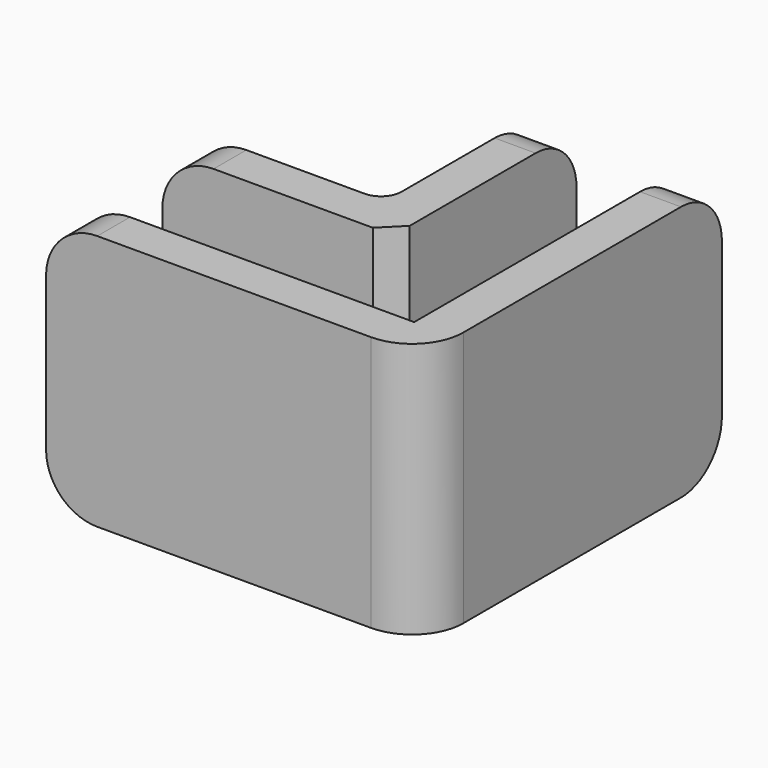
from build123d import *
from build123d import SkipClean  # not in build123d's __all__

# Parameters (mm, degrees)
F1_DEPTH       = 2
F2_DEPTH       = 25
F3_T1_DEPTH    = 29
F3_T3_DEPTH    = 29
F3_T5_DEPTH    = 29
F3_T7_DEPTH    = 29
F3_T9_DEPTH    = 43.2
F3_T11_DEPTH   = 43.2
F3_T13_DEPTH   = 50
F4_R           = 2
F5_SIZE        = 2
F7_D           = 3.3
F7_CSINK_D     = 6
F7_CSINK_ANGLE = 90


# Not quite as in the source:
# - a fillet or chamfer that OpenCascade refuses, or shapes differently, is made with other operations: its cross-section is extruded or revolved along the edge and cut away or added
# - a feature names something its author has since deleted; it is built from what else it names


with BuildPart() as f1:
    # F0 (on Top) → F1 (new body)
    with BuildSketch(Plane.XY):
        Polygon((5.1, 0), (5.1, 10.2), (5.1, 32.5735770881), (-5.1, 32.5735770881), (-5.1, 10.2), (-27.6520505063, 10.2), (-27.6520505063, 0), (0, 0), align=None)
        Polygon((5.1, 32.5735770881), (5.1, 10.2), (5.1, 0), (0, 0), (-27.6520505063, 0), (-27.6520505063, -4), (0, -4), (9.1, -4), (9.1, 32.5735770881), align=None)
        Polygon((-5.1, 10.2), (-5.1, 32.5735770881), (-9.1, 32.5735770881), (-9.1, 14.2), (-27.6520505063, 14.2), (-27.6520505063, 10.2), align=None)
    extrude(amount=F1_DEPTH)

    # F0 (on Top) → F2 (join)
    with BuildSketch(Plane.XY):
        Polygon((-5.1, 10.2), (-5.1, 32.5735770881), (-9.1, 32.5735770881), (-9.1, 14.2), (-27.6520505063, 14.2), (-27.6520505063, 10.2), align=None)
        Polygon((5.1, 32.5735770881), (5.1, 10.2), (5.1, 0), (0, 0), (-27.6520505063, 0), (-27.6520505063, -4), (0, -4), (9.1, -4), (9.1, 32.5735770881), align=None)
    extrude(amount=F2_DEPTH)

    # F3: fillet of radius 5 on 7 edges, made by hand

    # F3_s2 → F3_t1 (cut)
    with BuildSketch(Plane.XZ.offset(-12.5)):
        with BuildLine():
            ThreePointArc((-22.6520505063, 25), (-26.1875844123, 23.5355339059), (-27.6520505063, 20))
            Line((-27.6520505063, 20), (-27.6520505063, 25))
            Line((-27.6520505063, 25), (-22.6520505063, 25))
        make_face()
    extrude(amount=F3_T1_DEPTH, mode=Mode.SUBTRACT)

    # F3_s4 → F3_t3 (cut)
    with BuildSketch(Plane.XZ.offset(-26.7)):
        with BuildLine():
            ThreePointArc((-22.6520505063, 25), (-26.1875844123, 23.5355339059), (-27.6520505063, 20))
            Line((-27.6520505063, 20), (-27.6520505063, 25))
            Line((-27.6520505063, 25), (-22.6520505063, 25))
        make_face()
    extrude(amount=F3_T3_DEPTH, mode=Mode.SUBTRACT)

    # F3_s6 → F3_t5 (cut)
    with BuildSketch(Plane.YZ.offset(-21.6)):
        with BuildLine():
            ThreePointArc((27.5735770881, 25), (31.1091109941, 23.5355339059), (32.5735770881, 20))
            Line((32.5735770881, 20), (32.5735770881, 25))
            Line((32.5735770881, 25), (27.5735770881, 25))
        make_face()
    extrude(amount=F3_T5_DEPTH, mode=Mode.SUBTRACT)

    # F3_s8 → F3_t7 (cut)
    with BuildSketch(Plane.YZ.offset(-7.4)):
        with BuildLine():
            ThreePointArc((32.5735770881, 20), (31.1091109941, 23.5355339059), (27.5735770881, 25))
            Line((27.5735770881, 25), (32.5735770881, 25))
            Line((32.5735770881, 25), (32.5735770881, 20))
        make_face()
    with SkipClean():  # cleaning this boolean's faces spoils the solid; the shape is the same uncleaned
        extrude(amount=F3_T7_DEPTH, mode=Mode.SUBTRACT)

    # F3_s10 → F3_t9 (cut)
    with BuildSketch(Plane.XZ.offset(-26.7)):
        with BuildLine():
            ThreePointArc((-22.6520505063, 0), (-26.1875844123, 1.4644660941), (-27.6520505063, 5))
            Line((-27.6520505063, 5), (-27.6520505063, 0))
            Line((-27.6520505063, 0), (-22.6520505063, 0))
        make_face()
    extrude(amount=F3_T9_DEPTH, mode=Mode.SUBTRACT)

    # F3_s12 → F3_t11 (cut)
    with BuildSketch(Plane.YZ.offset(-21.6)):
        with BuildLine():
            ThreePointArc((27.5735770881, 0), (31.1091109941, 1.4644660941), (32.5735770881, 5))
            Line((32.5735770881, 5), (32.5735770881, 0))
            Line((32.5735770881, 0), (27.5735770881, 0))
        make_face()
    extrude(amount=F3_T11_DEPTH, mode=Mode.SUBTRACT)

    # F3_s14 → F3_t13 (cut)
    with BuildSketch(Plane.XY.offset(-12.5)):
        with BuildLine():
            ThreePointArc((4.1, -4), (7.6355339059, -2.5355339059), (9.1, 1))
            Line((9.1, 1), (9.1, -4))
            Line((9.1, -4), (4.1, -4))
        make_face()
    extrude(amount=F3_T13_DEPTH, mode=Mode.SUBTRACT)

    # F4
    f4_edges = [f1.edges().sort_by_distance(p)[0] for p in [
        (-9.1, 14.2, 12.5),
    ]]
    fillet(f4_edges, radius=F4_R)

    # F5
    f5_edges = [f1.edges().sort_by_distance(p)[0] for p in [
        (-5.1, 10.2, 13.5),
    ]]
    chamfer(f5_edges, length=F5_SIZE)

    # F7 (through all)
    with Locations(Plane(origin=(0, 0, 0), x_dir=(1, 0, 0), z_dir=(0, 0, -1))):
        with Locations((-15, -5.1), (0, -20.1)):
            CounterSinkHole(F7_D / 2, F7_CSINK_D / 2, counter_sink_angle=F7_CSINK_ANGLE)


solid = f1.part
